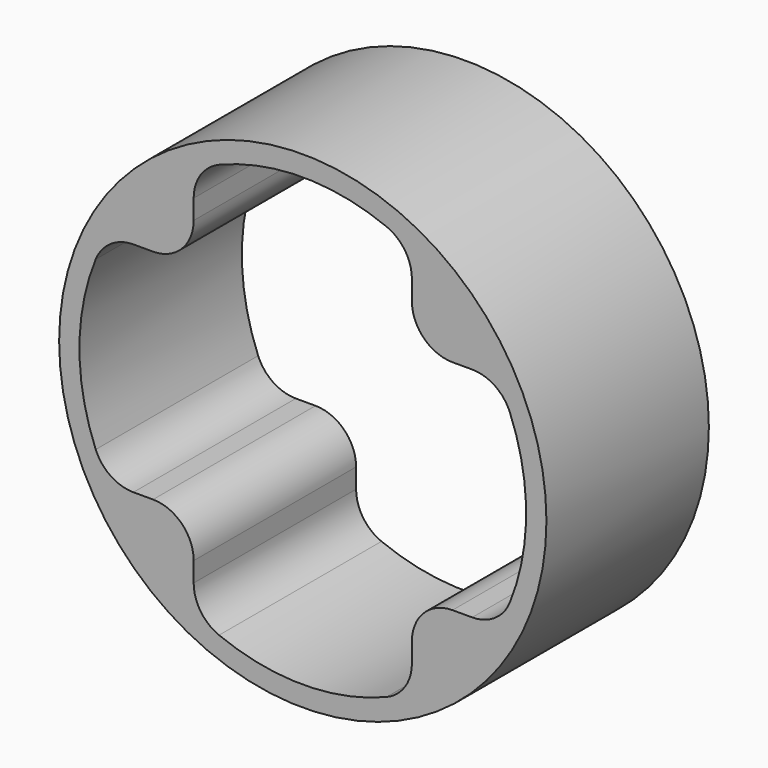
from build123d import *

# Parameters (mm, degrees)
F0_R     = 30
F0_R_2   = 27.5
F1_DEPTH = 25
F3_DEPTH = 25
F4_R     = 5


with BuildPart() as f1:
    # F0 (on Front) → F1 (new body)
    with BuildSketch(Plane.XZ):
        Circle(F0_R)
        Circle(F0_R_2, mode=Mode.SUBTRACT)
    extrude(amount=F1_DEPTH)

    # F2 (on Front) → F3 (join)
    with BuildSketch(Plane.XZ):
        with BuildLine():
            Line((-24.4350288425, 13.4350288425), (-18.4350288425, 13.4350288425))
            ThreePointArc((-18.4350288425, 13.4350288425), (-14.8994949366, 14.8994949366), (-13.4350288425, 18.4350288425))
            Line((-13.4350288425, 18.4350288425), (-13.4350288425, 24.4350288425))
            ThreePointArc((-13.4350288425, 24.4350288425), (-19.7176397489, 19.7176397489), (-24.4350288425, 13.4350288425))
        make_face()
        with BuildLine():
            ThreePointArc((18.4350288425, -13.4350288425), (14.8994949366, -14.8994949366), (13.4350288425, -18.4350288425))
            Line((13.4350288425, -18.4350288425), (13.4350288425, -24.4350288425))
            ThreePointArc((13.4350288425, -24.4350288425), (19.7176397489, -19.7176397489), (24.4350288425, -13.4350288425))
            Line((24.4350288425, -13.4350288425), (18.4350288425, -13.4350288425))
        make_face()
        with BuildLine():
            ThreePointArc((13.4350288425, 18.4350288425), (14.8994949366, 14.8994949366), (18.4350288425, 13.4350288425))
            Line((18.4350288425, 13.4350288425), (24.4350288425, 13.4350288425))
            ThreePointArc((24.4350288425, 13.4350288425), (19.7176397489, 19.7176397489), (13.4350288425, 24.4350288425))
            Line((13.4350288425, 24.4350288425), (13.4350288425, 18.4350288425))
        make_face()
        with BuildLine():
            Line((-13.4350288425, -24.4350288425), (-13.4350288425, -18.4350288425))
            ThreePointArc((-13.4350288425, -18.4350288425), (-14.8994949366, -14.8994949366), (-18.4350288425, -13.4350288425))
            Line((-18.4350288425, -13.4350288425), (-24.4350288425, -13.4350288425))
            ThreePointArc((-24.4350288425, -13.4350288425), (-19.7176397489, -19.7176397489), (-13.4350288425, -24.4350288425))
        make_face()
    extrude(amount=F3_DEPTH)

    # F4
    f4_edges = [f1.edges().sort_by_distance(p)[0] for p in [
        (-13.435029, -12.5, 23.994791),
        (-23.994791, -12.5, 13.435029),
        (-23.994791, -12.5, -13.435029),
        (-13.435029, -12.5, -23.994791),
        (13.435029, -12.5, 23.994791),
        (23.994791, -12.5, 13.435029),
        (13.435029, -12.5, -23.994791),
        (23.994791, -12.5, -13.435029),
    ]]
    fillet(f4_edges, radius=F4_R)


solid = f1.part
